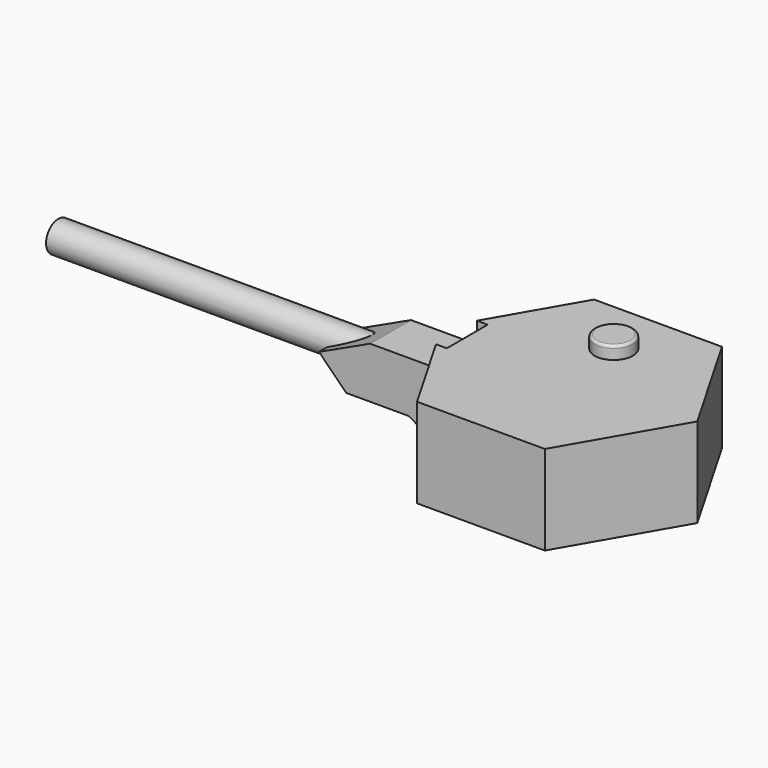
from build123d import *

# Parameters (mm, degrees)
F1_DEPTH    = 35
F2_R        = 7.5
F3_DEPTH    = 5
F4_R        = 1
F5_W        = 20
F5_H        = 20
F6_DEPTH    = 35.001
F7_T        = 7.5
F7_T3_DEPTH = 50
F10_DEPTH   = 10
F9_R        = 6
F11_DEPTH   = 200


# Not quite as in the source:
# - a shell that OpenCascade refuses in one call is made with other operations: the cavity is built on its own and cut out


with BuildPart() as f1:
    # F0 (on Top) → F1 (new body)
    with BuildSketch(Plane.XY):
        Polygon((25, 43.3012701892), (-25, 43.3012701892), (-50, 0), (-25, -43.3012701892), (25, -43.3012701892), (50, 0), align=None)
    extrude(amount=F1_DEPTH)

    # F2 (on face) → F3 (join)
    with BuildSketch(Plane.XY.offset(35)):
        with Locations((0, 21.6506350946)):
            Circle(F2_R)
    extrude(amount=F3_DEPTH)

    # F4
    f4_edges = [f1.edges().sort_by_distance(p)[0] for p in [
        (-7.5, 21.650635, 40),
    ]]
    fillet(f4_edges, radius=F4_R)

    # F5 (on face) → F6 (cut, through all)
    with BuildSketch(Plane.XY.offset(35)):
        with Locations((-50, 0)):
            Rectangle(F5_W, F5_H)
    extrude(amount=-F6_DEPTH, mode=Mode.SUBTRACT)

    # F7: shell of thickness 7.5, made by hand


with BuildPart() as f7_core1:
    # F7_t2: copy of F1
    add(f1.part)

    # the walls: a layer under each face that stays
    f7_faces = [f7_core1.faces().sort_by_distance(p)[0] for p in [
        (2.8867513459, 0, 35),
        (0, 21.6506350946, 40),
        (37.5, 21.6506350946, 17.5),
        (37.5, -21.6506350946, 17.5),
        (0, -43.3012701892, 17.5),
        (-34.6132486541, -26.6506350946, 17.5),
        (-42.1132486541, -10, 17.5),
        (-40, 0, 17.5),
        (-42.1132486541, 10, 17.5),
        (-34.6132486541, 26.6506350946, 17.5),
        (0, 43.3012701892, 17.5),
    ]]
    thicken(f7_faces, amount=-F7_T, mode=Mode.SUBTRACT)

    # F7_s4 → F7_t3 (cut)
    with BuildSketch(Plane.XY.offset(-7.5)):
        Polygon((-40.075, -9.925), (-40, -17.5), (-32.5, -17.5), (-32.5, -10), align=None)
        Polygon((-40.075, 9.925), (-32.5, 10), (-32.5, 17.5), (-40, 17.5), align=None)
    extrude(amount=F7_T3_DEPTH, mode=Mode.SUBTRACT)

    # F7_s5 → F7_t6 (revolve, cut)
    with BuildSketch(Plane.XZ.offset(-21.6506350946)):
        Polygon((7.575, 35.075), (0, 35), (0, 27.5), (7.5, 27.5), align=None)
    revolve(axis=Axis((0, 21.6506350946, 35), (0, 0, 1)), mode=Mode.SUBTRACT)


with BuildPart() as f1_1:
    add(f1.part)

    # what is left inside the walls is the cavity
    f7_cavity = [f7_core1.part.solids().sort_by_distance(p)[0] for p in [
        (4.419873, -11.933757, 27.425),
    ]]
    add(f7_cavity, mode=Mode.SUBTRACT)

    # F8 (on Front) → F10 (join, symmetric)
    with BuildSketch(Plane.XZ):
        Polygon((-10, 6.8261531631), (-10, 26.8261531631), (-70, 26.8261531631), (-90, 17.5), (-79.3261531631, 6.8261531631), (-54.9282032303, 6.8261531631), (-49.7320508076, 3.8261531631), (-48, 6.8261531631), align=None)
    extrude(amount=F10_DEPTH, both=True)

    # F9 (on Right) → F11 (join)
    with BuildSketch(Plane.YZ):
        with Locations((0, 17.5)):
            Circle(F9_R)
    extrude(amount=-F11_DEPTH)


solid = f1_1.part
